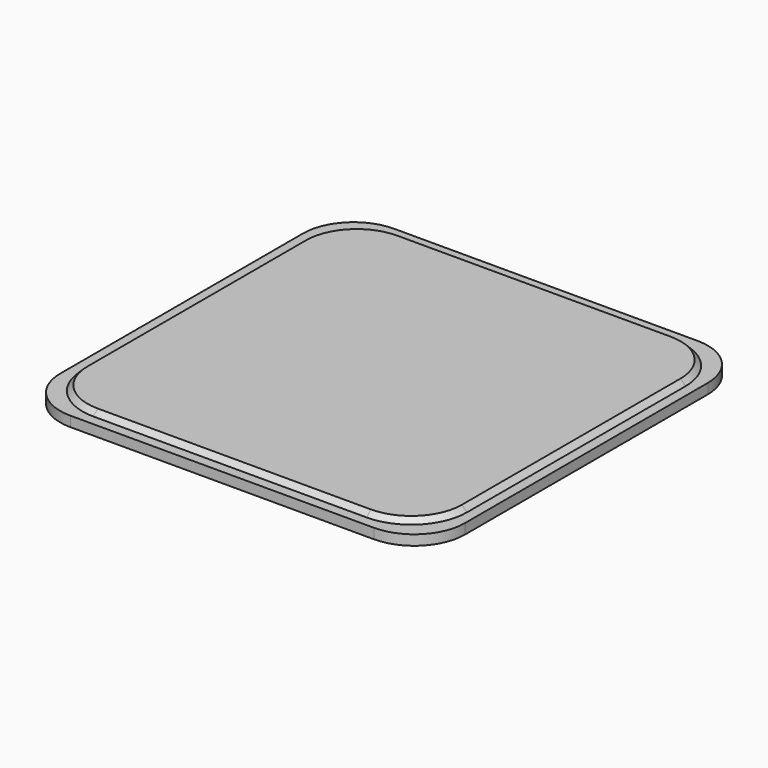
from build123d import *

# Parameters (mm, degrees)
F1_DEPTH = 2.54
F3_DEPTH = 1.27
F5_DEPTH = 1.27
F6_SIZE  = 1.26999
F7_SIZE  = 1.26999


# Not quite as in the source:
# - a fillet or chamfer is up to 0.001 mm smaller than in the source, because OpenCascade refuses the exact size


with BuildPart() as f1:
    # F0 (on Top) → F1 (new body)
    with BuildSketch(Plane.XY):
        with BuildLine():
            ThreePointArc((50.8, 38.1), (47.0802561211, 47.0802561211), (38.1, 50.8))
            Line((38.1, 50.8), (-38.1, 50.8))
            ThreePointArc((-38.1, 50.8), (-47.0802561211, 47.0802561211), (-50.8, 38.1))
            Line((-50.8, 38.1), (-50.8, -38.1))
            ThreePointArc((-50.8, -38.1), (-47.0802561211, -47.0802561211), (-38.1, -50.8))
            Line((-38.1, -50.8), (38.1, -50.8))
            ThreePointArc((38.1, -50.8), (47.0802561211, -47.0802561211), (50.8, -38.1))
            Line((50.8, -38.1), (50.8, 38.1))
        make_face()
    extrude(amount=F1_DEPTH)

    # F2 (on face) → F3 (join)
    with BuildSketch(Plane(origin=(0, 0, 0), x_dir=(1, 0, 0), z_dir=(0, 0, -1))):
        with BuildLine():
            Line((-38.1, -50.8), (38.1, -50.8))
            ThreePointArc((38.1, -50.8), (47.0802561211, -47.0802561211), (50.8, -38.1))
            Line((50.8, -38.1), (50.8, 38.1))
            ThreePointArc((50.8, 38.1), (47.0802561211, 47.0802561211), (38.1, 50.8))
            Line((38.1, 50.8), (-38.1, 50.8))
            ThreePointArc((-38.1, 50.8), (-47.0802561211, 47.0802561211), (-50.8, 38.1))
            Line((-50.8, 38.1), (-50.8, -38.1))
            ThreePointArc((-50.8, -38.1), (-47.0802561211, -47.0802561211), (-38.1, -50.8))
        make_face()
        with BuildLine():
            Line((-34.925, 47.625), (34.925, 47.625))
            ThreePointArc((34.925, 47.625), (43.9052561211, 43.9052561211), (47.625, 34.925))
            Line((47.625, 34.925), (47.625, -34.925))
            ThreePointArc((47.625, -34.925), (43.9052561211, -43.9052561211), (34.925, -47.625))
            Line((34.925, -47.625), (-34.925, -47.625))
            ThreePointArc((-34.925, -47.625), (-43.9052561211, -43.9052561211), (-47.625, -34.925))
            Line((-47.625, -34.925), (-47.625, 34.925))
            ThreePointArc((-47.625, 34.925), (-43.9052561211, 43.9052561211), (-34.925, 47.625))
        make_face(mode=Mode.SUBTRACT)
    extrude(amount=F3_DEPTH)

    # F4 (on face) → F5 (cut)
    with BuildSketch(Plane.XY.offset(2.54)):
        with BuildLine():
            Line((50.8, -38.1), (50.8, 38.1))
            ThreePointArc((50.8, 38.1), (47.0802561211, 47.0802561211), (38.1, 50.8))
            Line((38.1, 50.8), (-38.1, 50.8))
            ThreePointArc((-38.1, 50.8), (-47.0802561211, 47.0802561211), (-50.8, 38.1))
            Line((-50.8, 38.1), (-50.8, -38.1))
            ThreePointArc((-50.8, -38.1), (-47.0802561211, -47.0802561211), (-38.1, -50.8))
            Line((-38.1, -50.8), (38.1, -50.8))
            ThreePointArc((38.1, -50.8), (47.0802561211, -47.0802561211), (50.8, -38.1))
        make_face()
        with BuildLine():
            ThreePointArc((46.99, -34.29), (43.2702561211, -43.2702561211), (34.29, -46.99))
            Line((34.29, -46.99), (-34.29, -46.99))
            ThreePointArc((-34.29, -46.99), (-43.2702561211, -43.2702561211), (-46.99, -34.29))
            Line((-46.99, -34.29), (-46.99, 34.29))
            ThreePointArc((-46.99, 34.29), (-43.2702561211, 43.2702561211), (-34.29, 46.99))
            Line((-34.29, 46.99), (34.29, 46.99))
            ThreePointArc((34.29, 46.99), (43.2702561211, 43.2702561211), (46.99, 34.29))
            Line((46.99, 34.29), (46.99, -34.29))
        make_face(mode=Mode.SUBTRACT)
    extrude(amount=-F5_DEPTH, mode=Mode.SUBTRACT)

    # F6 (size 1.27 in the source; OpenCascade refuses exactly that, so slightly less here)
    f6_edges = [f1.edges().sort_by_distance(p)[0] for p in [
        (0, 46.99, 1.27),
        (-43.270256, 43.270256, 1.27),
        (-46.99, 0, 1.27),
        (-43.270256, -43.270256, 1.27),
    ]]
    chamfer(f6_edges, length=F6_SIZE)

    # F7 (size 1.27 in the source; OpenCascade refuses exactly that, so slightly less here)
    f7_edges = [f1.edges().sort_by_distance(p)[0] for p in [
        (-43.905256, -43.905256, 0),
        (-47.625, 0, 0),
        (-43.905256, 43.905256, 0),
        (0, 47.625, 0),
        (43.905256, 43.905256, 0),
        (47.625, 0, 0),
        (43.905256, -43.905256, 0),
        (0, -47.625, 0),
    ]]
    chamfer(f7_edges, length=F7_SIZE)


solid = f1.part
